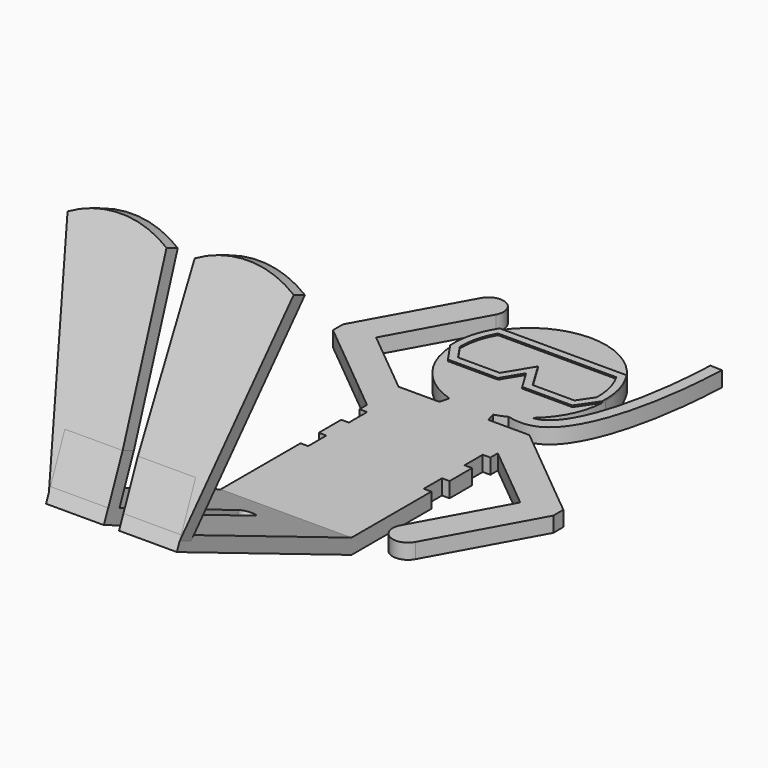
from build123d import *

# Parameters (mm, degrees)
F1_DEPTH = 2
F3_DEPTH = 17.200789751
F4_W     = 1
F4_H     = 2
F5_DEPTH = 25
F7_DEPTH = 2
F9_DEPTH = 0.2


# Not quite as in the source:
# - the dataset's text gives a spline's control points without its knots; the knots are read off the source's solid
# - a feature names something its author has since deleted; it is built from what else it names


with BuildPart() as f1:
    # F0 (on Top) → F1 (new body)
    with BuildSketch(Plane.XY):
        with BuildLine():
            ThreePointArc((6.4629719502, -7.6308579839), (9.0727537028, -4.2053704057), (10, 0))
            ThreePointArc((10, 0), (-5.9694275413, 8.0228383275), (-2.8731869657, -9.5783504143))
            Line((-2.8731869657, -9.5783504143), (0, 0))
            Line((0, 0), (1.8618540828, -6.2738101865))
            add(Edge.make_bspline(
                [(1.8618540828, -6.2738101865), (1.9794198127, -6.3341629295), (2.5732776532, -6.6333178765), (3.6057370778, -7.0964112527), (4.8687885055, -7.50576435), (5.8045739388, -7.6494945297), (6.2976751035, -7.6438504545), (6.4629719502, -7.6308579839)],
                knots=[0.0471973375, 0.0471973375, 0.0471973375, 0.0471973375, 0.0625, 0.125, 0.1875, 0.25, 0.2838293075, 0.2838293075, 0.2838293075, 0.2838293075], degree=3))
        make_face()
        with BuildLine():
            Line((0, 0), (-2.8731869657, -9.5783504143))
            ThreePointArc((-2.8731869657, -9.5783504143), (-0.0146952719, -9.9999892024), (2.8450232941, -9.5867534888))
            Line((2.8450232941, -9.5867534888), (2.4577875555, -8.2819017585))
            Line((2.4577875555, -8.2819017585), (1.8618540828, -6.2738101865))
            Line((1.8618540828, -6.2738101865), (0, 0))
        make_face()
        with BuildLine():
            ThreePointArc((2.8450232941, -9.5867534888), (-0.0146952719, -9.9999892024), (-2.8731869657, -9.5783504143))
            Line((-2.8731869657, -9.5783504143), (-3.241058439, -10.8047244445))
            Line((-3.241058439, -10.8047244445), (3.2064757654, -10.8047244445))
            Line((3.2064757654, -10.8047244445), (2.8450232941, -9.5867534888))
        make_face()
        with BuildLine():
            add(Edge.make_bspline(
                [(6.4629719502, -7.6308579839), (6.6030627596, -7.619846729), (6.8840296576, -7.5803052276), (7.2792450589, -7.4693493545), (7.6665868261, -7.2958798164), (8.0522350381, -7.0483493763), (8.4601010219, -6.700195356), (8.8775961576, -6.2496121629), (9.4379128784, -5.5115962551), (10.1252991034, -4.3405271139), (10.8897039738, -2.5813381399), (11.5728725961, -0.5166619682), (12.3603130252, 2.5826938425), (13.095778184, 6.9972675513), (13.399766994, 10.8869404738), (13.4782410246, 12.8689533823)],
                knots=[0.2838293075, 0.2838293075, 0.2838293075, 0.2838293075, 0.3125, 0.34375, 0.375, 0.40625, 0.4375, 0.46875, 0.5, 0.5625, 0.625, 0.6875, 0.75, 0.875, 1, 1, 1, 1], degree=3))
            ThreePointArc((6.4629719502, -7.6308579839), (5.4847517485, -8.3616683896), (4.4247539743, -8.9678064356))
            add(Edge.make_bspline(
                [(4.4247539743, -8.9678064356), (5.941531364, -9.347351876), (11.7155314673, -9.1561084525), (14.6416607546, 2.8636422945), (15.0353610516, 12.807302177)],
                knots=[0.1854268528, 0.1854268528, 0.1854268528, 0.1854268528, 0.3850411547, 1, 1, 1, 1], degree=3))
            Line((15.0353610516, 12.807302177), (13.4782410246, 12.8689533823))
        make_face()
        with BuildLine():
            ThreePointArc((4.4247539743, -8.9678064356), (5.4847517485, -8.3616683896), (6.4629719502, -7.6308579839))
            add(Edge.make_bspline(
                [(1.8618540828, -6.2738101865), (1.9794198127, -6.3341629295), (2.5732776532, -6.6333178765), (3.6057370778, -7.0964112527), (4.8687885055, -7.50576435), (5.8045739388, -7.6494945297), (6.2976751035, -7.6438504545), (6.4629719502, -7.6308579839)],
                knots=[0.0471973375, 0.0471973375, 0.0471973375, 0.0471973375, 0.0625, 0.125, 0.1875, 0.25, 0.2838293075, 0.2838293075, 0.2838293075, 0.2838293075], degree=3))
            Line((1.8618540828, -6.2738101865), (2.4577875555, -8.2819017585))
            add(Edge.make_bspline(
                [(2.4577875555, -8.2819017585), (3.1280804798, -8.5721149462), (3.7854626045, -8.8078356145), (4.4247539743, -8.9678064356)],
                knots=[0.1012934121, 0.1012934121, 0.1012934121, 0.1012934121, 0.1854268528, 0.1854268528, 0.1854268528, 0.1854268528], degree=3))
        make_face()
        with BuildLine():
            Line((2.4577875555, -8.2819017585), (2.8450232941, -9.5867534888))
            ThreePointArc((2.8450232941, -9.5867534888), (3.6480390961, -9.3108437186), (4.4247539743, -8.9678064356))
            add(Edge.make_bspline(
                [(2.4577875555, -8.2819017585), (3.1280804798, -8.5721149462), (3.7854626045, -8.8078356145), (4.4247539743, -8.9678064356)],
                knots=[0.1012934121, 0.1012934121, 0.1012934121, 0.1012934121, 0.1854268528, 0.1854268528, 0.1854268528, 0.1854268528], degree=3))
        make_face()
        Polygon((3.2064757654, -10.8047244445), (-3.241058439, -10.8047244445), (-8.6003948755, -10.8047244445), (-8.6003948755, -15.9862233672), (-8.6003948755, -17.2114234168), (-7.6003948755, -17.2114234168), (-7.6003948755, -20.2114234168), (-8.6003948755, -20.2114234168), (-8.6003948755, -23.9146029156), (-7.6003948755, -23.9146029156), (-7.6003948755, -26.9146029156), (-8.6003948755, -26.9146029156), (-8.6003948755, -40.0244813867), (8.6003948755, -40.0244813867), (8.6003948755, -26.9146029156), (7.6003948755, -26.9146029156), (7.6003948755, -23.9146029156), (8.6003948755, -23.9146029156), (8.6003948755, -20.2114234168), (7.6003948755, -20.2114234168), (7.6003948755, -17.2114234168), (8.6003948755, -17.2114234168), (8.6003948755, -15.9862233672), (8.6003948755, -10.8047244445), align=None)
        Polygon((-8.6003948755, -15.9862233672), (-8.6003948755, -10.8047244445), (-11.7467804993, -13.3954739058), align=None)
        with BuildLine():
            Line((-11.7467804993, -13.3954739058), (-8.6003948755, -10.8047244445))
            Line((-8.6003948755, -10.8047244445), (-17.2348651583, -3.6950589713))
            Line((-17.2348651583, -3.6950589713), (-10.8148216824, 7.9533712388))
            ThreePointArc((-10.8148216824, 7.9533712388), (-11.6010166189, 10.6703360015), (-14.3179813816, 9.884141065))
            Line((-14.3179813816, 9.884141065), (-21.7172442848, -3.5409701289))
            Line((-21.7172442848, -3.5409701289), (-21.7148243129, -5.1877374014))
            Line((-21.7148243129, -5.1877374014), (-11.7467804993, -13.3954739058))
        make_face()
        with BuildLine():
            Line((21.7148243129, -21.6032104103), (8.6003948755, -10.8047244445))
            Line((8.6003948755, -10.8047244445), (8.6003948755, -15.9862233672))
            Line((8.6003948755, -15.9862233672), (17.2348651583, -23.0958888404))
            Line((17.2348651583, -23.0958888404), (10.8148216824, -34.7443190505))
            ThreePointArc((10.8148216824, -34.7443190505), (11.6010166189, -37.4612838132), (14.3179813816, -36.6750888767))
            Line((14.3179813816, -36.6750888767), (21.7172442848, -23.2499776828))
            Line((21.7172442848, -23.2499776828), (21.7148243129, -21.6032104103))
        make_face()
    extrude(amount=F1_DEPTH)

    # F2 (on face) → F3 (join, through all)
    with BuildSketch(Plane.YZ.offset(8.6003948755)):
        Polygon((-40.0244813867, 0), (-40.0244813867, 2), (-66.176410403, 12.9284200062), (-66.8879257534, 11.2257494531), align=None)
        Polygon((-66.8879257534, 11.2257494531), (-66.176410403, 12.9284200062), (-68.0217670369, 13.6995612992), (-68.7332823873, 11.9968907461), align=None)
        Polygon((-68.0217670369, 13.6995612992), (-66.176410403, 12.9284200062), (-63.8033605813, 18.6071759886), (-65.6487172152, 19.3783172816), align=None)
    extrude(amount=-F3_DEPTH)

    # F4 (on face) → F5 (cut)
    with BuildSketch(Plane(origin=(0, -2.8656632843, -6.8575899128), x_dir=(1, 0, 0), z_dir=(0, 0.3855706465, 0.9226783169))):
        with Locations((-0.5, -67.044358232)):
            Rectangle(F4_W, F4_H)
        with BuildLine():
            Line((1, -68.044358232), (0, -68.044358232))
            Line((0, -68.044358232), (-1, -68.044358232))
            Line((-1, -68.044358232), (-1, -69.7565637529))
            ThreePointArc((-1, -69.7565637529), (0, -70.7565637529), (1, -69.7565637529))
            Line((1, -69.7565637529), (1, -68.044358232))
        make_face()
        with Locations((0.5, -67.044358232)):
            Rectangle(F4_W, F4_H)
        with BuildLine():
            Line((-1, -66.044358232), (0, -66.044358232))
            Line((0, -66.044358232), (1, -66.044358232))
            Line((1, -66.044358232), (1, -44.7565637529))
            ThreePointArc((1, -44.7565637529), (0, -43.7565637529), (-1, -44.7565637529))
            Line((-1, -44.7565637529), (-1, -66.044358232))
        make_face()
    extrude(amount=-F5_DEPTH, mode=Mode.SUBTRACT)

    # F6 (on face) → F7 (join)
    with BuildSketch(Plane(origin=(0, -62.7830539309, 26.2359071944), x_dir=(1, 0, 0), z_dir=(0, -0.9226783169, 0.3855706465))):
        with BuildLine():
            ThreePointArc((-1.8515158445, 14.0382554382), (-8.3589539863, 15.7649961788), (-14.8663921282, 14.0382554382))
            Line((-14.8663921282, 14.0382554382), (-1.8515158445, 14.0382554382))
        make_face()
        Polygon((1, -15.4322651642), (8.6003948755, -15.4322651642), (8.6003948755, -14.2483813688), (8.6003948755, -7.4322651642), (1, -7.4322651642), align=None)
        with BuildLine():
            Line((8.6003948755, -7.4322651642), (8.6003948755, -14.2483813688))
            Line((8.6003948755, -14.2483813688), (14.8663921282, 14.0382554382))
            ThreePointArc((14.8663921282, 14.0382554382), (8.3589539863, 15.7649961788), (1.8515158445, 14.0382554382))
            Line((1.8515158445, 14.0382554382), (1, -7.4322651642))
            Line((1, -7.4322651642), (8.6003948755, -7.4322651642))
        make_face()
        Polygon((-8.6003948755, -7.4322651642), (-1, -7.4322651642), (-1.8515158445, 14.0382554382), (-14.8663921282, 14.0382554382), (-8.6003948755, -14.2483813688), align=None)
    extrude(amount=-F7_DEPTH)

    # F8 (on face) → F9 (join)
    with BuildSketch(Plane.XY.offset(2)):
        with BuildLine():
            Line((8.3395420131, 5.5183366165), (-8.3395420131, 5.5183366165))
            ThreePointArc((-8.3395420131, 5.5183366165), (-9.6548741312, 2.6044971704), (-9.9834241522, -0.575536443))
            Line((-9.9834241522, -0.575536443), (-8.1826943192, -3.206660389))
            Line((-8.1826943192, -3.206660389), (-1.5899471466, -3.206660389))
            Line((-1.5899471466, -3.206660389), (0, -0.575536443))
            Line((0, -0.575536443), (1.5899471466, -3.206660389))
            Line((1.5899471466, -3.206660389), (8.1826943192, -3.206660389))
            Line((8.1826943192, -3.206660389), (9.9834241522, -0.575536443))
            ThreePointArc((9.9834241522, -0.575536443), (9.6548741312, 2.6044971704), (8.3395420131, 5.5183366165))
        make_face()
        with BuildLine():
            ThreePointArc((-8.9966146265, -0.2468304304), (-8.721852762, 2.2201991799), (-7.7836131854, 4.5183366165))
            Line((-7.7836131854, 4.5183366165), (7.7836131854, 4.5183366165))
            ThreePointArc((7.7836131854, 4.5183366165), (8.721852762, 2.2201991799), (8.9966146265, -0.2468304304))
            Line((8.9966146265, -0.2468304304), (7.6553154911, -2.206660389))
            Line((7.6553154911, -2.206660389), (2.1540632086, -2.206660389))
            Line((2.1540632086, -2.206660389), (0, 1.3579909904))
            Line((0, 1.3579909904), (-2.1540632086, -2.206660389))
            Line((-2.1540632086, -2.206660389), (-7.6553154911, -2.206660389))
            Line((-7.6553154911, -2.206660389), (-8.9966146265, -0.2468304304))
        make_face(mode=Mode.SUBTRACT)
    extrude(amount=F9_DEPTH)


solid = f1.part
